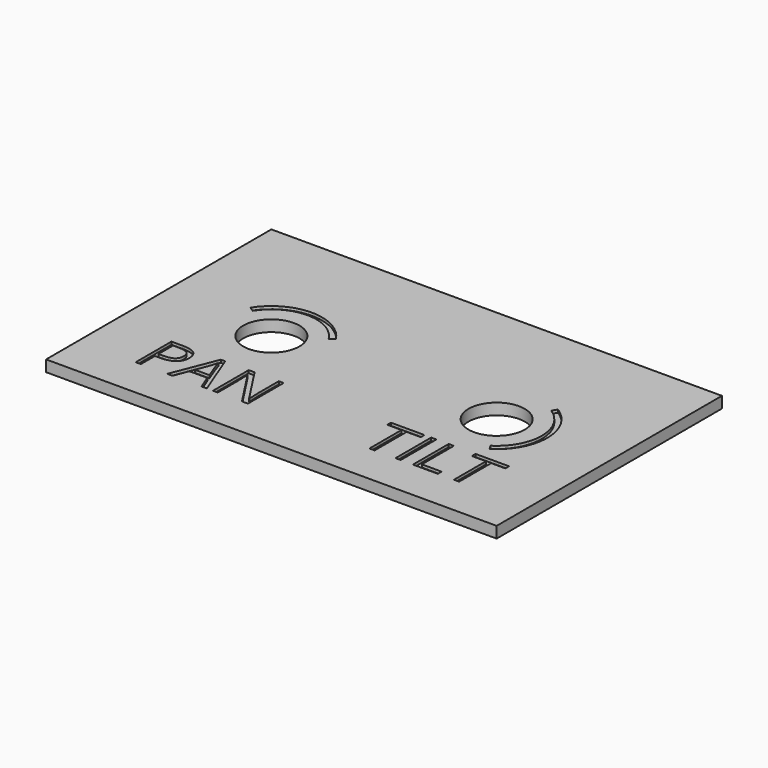
from build123d import *

# Parameters (mm, degrees)
F0_W         = 80
F0_H         = 50
F0_R         = 5
F1_DEPTH     = 2
F2_TEXT_SIZE = 11.1111111111
F3_DEPTH     = 0.5
F5_DEPTH     = 0.5


# Not quite as in the source:
# - Text() gives the source's letters only with a copy of the font that has no kerning and outlines rounded to 1/6400 em; it was checked with that copy


with BuildPart() as f1:
    # F0 (on Top) → F1 (new body)
    with BuildSketch(Plane.XY):
        Rectangle(F0_W, F0_H)
        with Locations((-20, 0)):
            Circle(F0_R, mode=Mode.SUBTRACT)
        with Locations((20, 0)):
            Circle(F0_R, mode=Mode.SUBTRACT)
    extrude(amount=F1_DEPTH)

    # F2 (on face) → F3 (cut)
    with BuildSketch(Plane.XY.offset(2)):
        with Locations((-30.8637152778, -17.8904977177)):
            Text('PAN', F2_TEXT_SIZE, font='Open Sans', text_align=(TextAlign.LEFT, TextAlign.BOTTOM))
        with Locations((9.1119791667, -17.8904977177)):
            Text('TILT', F2_TEXT_SIZE, font='Open Sans', text_align=(TextAlign.LEFT, TextAlign.BOTTOM))
    extrude(amount=-F3_DEPTH, mode=Mode.SUBTRACT)

    # F4 (on face) → F5 (cut)
    with BuildSketch(Plane.XY.offset(2)):
        with BuildLine():
            ThreePointArc((-26.7471315665, 4.2983968668), (-20, 8), (-13.2528684335, 4.2983968668))
            Line((-13.2528684335, 4.2983968668), (-12.4094769877, 4.8356964751))
            ThreePointArc((-12.4094769877, 4.8356964751), (-20, 9), (-27.5905230123, 4.8356964751))
            Line((-27.5905230123, 4.8356964751), (-26.7471315665, 4.2983968668))
        make_face()
        with BuildLine():
            ThreePointArc((24.2983968668, 6.7471315665), (28, 0), (24.2983968668, -6.7471315665))
            Line((24.2983968668, -6.7471315665), (24.8356964751, -7.5905230123))
            ThreePointArc((24.8356964751, -7.5905230123), (29, 0), (24.8356964751, 7.5905230123))
            Line((24.8356964751, 7.5905230123), (24.2983968668, 6.7471315665))
        make_face()
    extrude(amount=-F5_DEPTH, mode=Mode.SUBTRACT)


solid = f1.part
